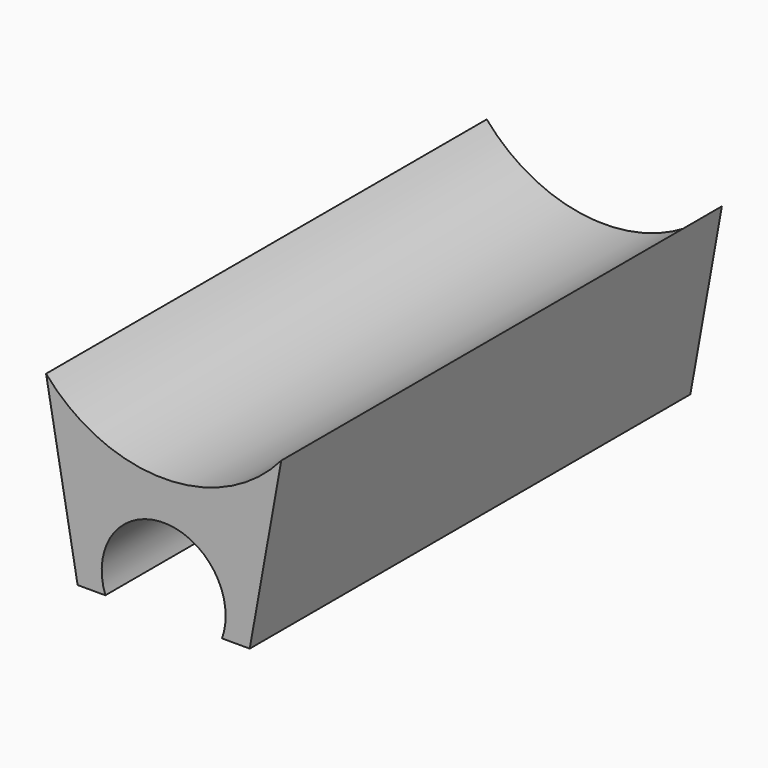
from build123d import *

# Parameters (mm, degrees)
F1_DEPTH = 50.8


# Not quite as in the source:
# - a feature names something its author has since deleted; it is built from what else it names


with BuildPart() as f1:
    # F0 (on Front) → F1 (new body)
    with BuildSketch(Plane.XZ):
        with BuildLine():
            Line((7.9375, -1.9304), (10.8458, 14.2875))
            ThreePointArc((10.8458, 14.2875), (0, 9.3006063571), (-10.8458, 14.2875))
            Line((-10.8458, 14.2875), (-7.9375, -1.9304))
            Line((-7.9375, -1.9304), (-5.3791059517, -1.9304))
            ThreePointArc((-5.3791059517, -1.9304), (-0.9797026298, 5.6304003194), (5.715, 0))
            ThreePointArc((5.715, 0), (5.6304003194, -0.9797026298), (5.3791059517, -1.9304))
            Line((5.3791059517, -1.9304), (7.9375, -1.9304))
        make_face()
    extrude(amount=F1_DEPTH)


solid = f1.part
